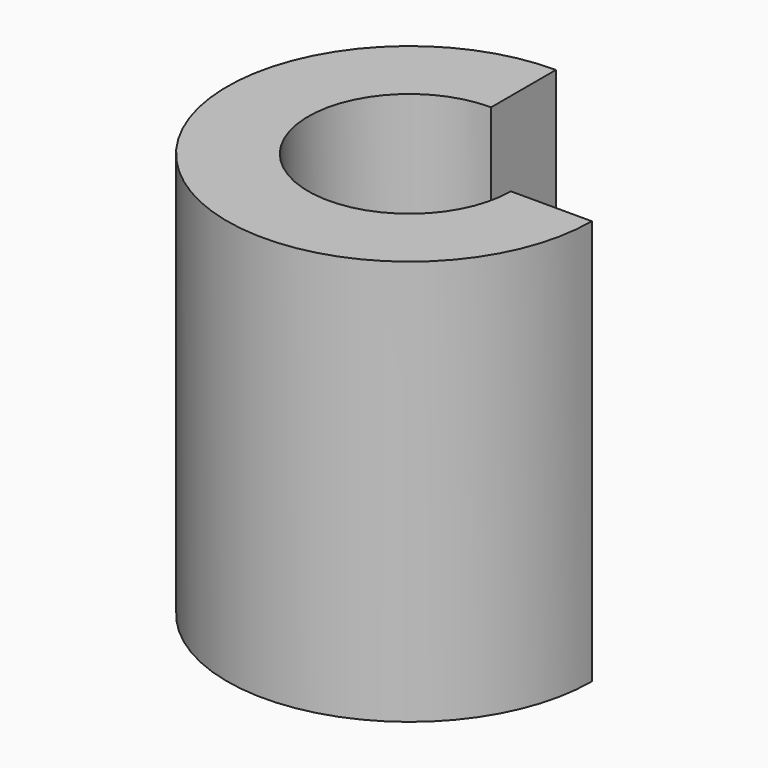
from build123d import *

# Parameters (mm, degrees)
F1_DEPTH = 10


# Not quite as in the source:
# - ends of sketch curves that miss each other by under 0.0002 mm in the source are joined


with BuildPart() as f1:
    # F0 (on Top) → F1 (new body)
    with BuildSketch(Plane.XY):
        with BuildLine():
            ThreePointArc((2.5, 0), (-1.767766953, -1.767766953), (0, 2.5))
            ThreePointArc((0, 2.5), (0.0073339568, 2.4999892426), (0.0146678504, 2.4999569705))
            Line((0.0146678504, 2.4999569705), (0.0146679766, 4.4999760944))
            ThreePointArc((0.0146679766, 4.4999760944), (-3.1871622092, -3.1767903696), (4.5, 0))
            Line((4.5, 0), (2.5, 0))
        make_face()
    extrude(amount=F1_DEPTH)


solid = f1.part
